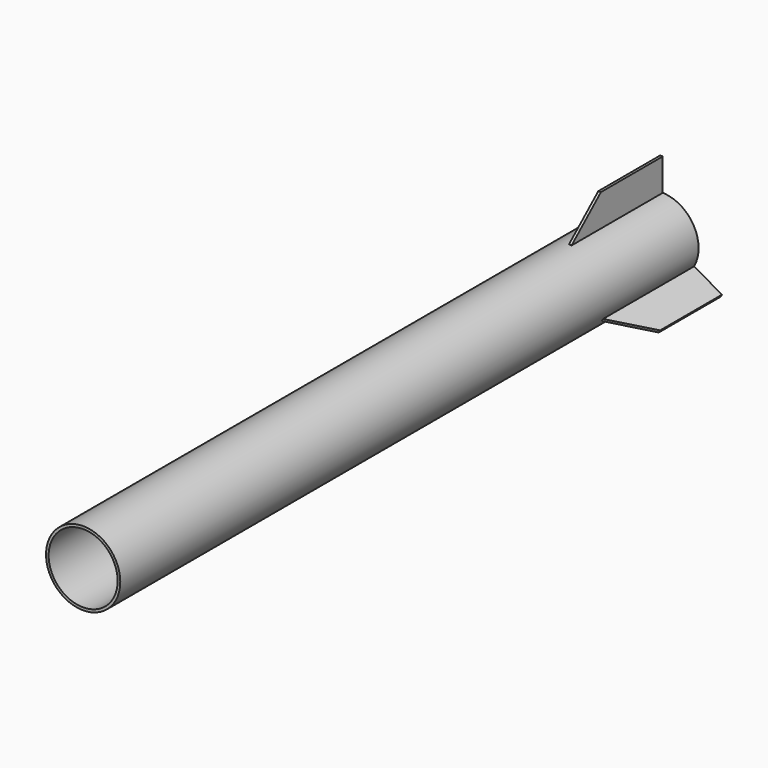
from build123d import *

# Parameters (mm, degrees)
F0_R     = 11.3
F0_R_2   = 10.5
F1_DEPTH = 220
F3_DEPTH = 0.4
F4_COUNT = 3


with BuildPart() as f1:
    # F0 (on Front) → F1 (new body)
    with BuildSketch(Plane.XZ):
        Circle(F0_R)
        Circle(F0_R_2, mode=Mode.SUBTRACT)
    extrude(amount=F1_DEPTH)


with BuildPart() as f3:
    # F2 (on Right) → F3 (new body, symmetric)
    with BuildSketch(Plane.YZ):
        Polygon((-35, 11.013663877), (0, 11.013663877), (0, 21.0248362273), (-23.5218461603, 21.0248362273), align=None)
    extrude(amount=F3_DEPTH, both=True)


with BuildPart() as f4_1:
    # F4: instance of F3
    add(f3.part.rotate(Axis((0, 0, 0), (0, 1, 0)), 1 * 360 / F4_COUNT))


with BuildPart() as f4_2:
    # F4: instance of F3
    add(f3.part.rotate(Axis((0, 0, 0), (0, 1, 0)), 2 * 360 / F4_COUNT))


solid = Compound([f1.part, f3.part, f4_1.part, f4_2.part])
